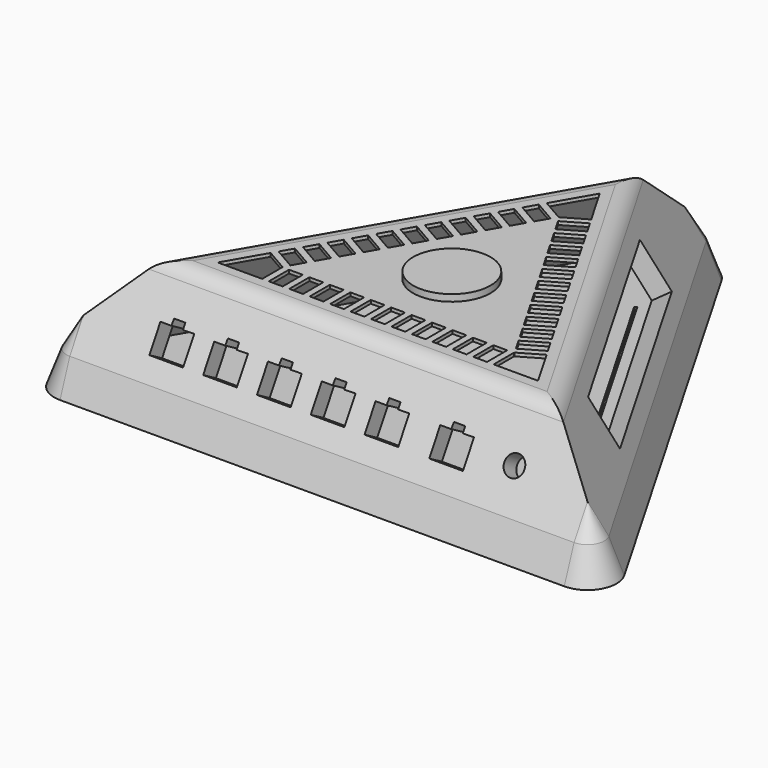
from build123d import *

# Parameters (mm, degrees)
F1_DEPTH      = 25
F1_TAPER      = 30
F1_DEPTH_BACK = 10
F1_TAPER_BACK = -20
F2_R          = 6
F3_R          = 11.5
F4_DEPTH      = 2
F6_R          = 7.5
F7_DEPTH      = 3
F8_R          = 32.5
F9_DEPTH      = 5
F10_R         = 3
F11_DEPTH     = 2
F13_DEPTH     = 5
F15_W         = 1.9796080887
F15_H         = 8.6034480482
F16_DEPTH     = 1
F17_DEPTH     = 10
F19_DEPTH     = 10
F21_DEPTH     = 24
F21_TAPER     = 30


with BuildPart() as f1:
    # F0 (on Top) → F1 (new body, two sides)
    with BuildSketch(Plane.XY) as f1_sk:
        with BuildLine():
            Line((-75, -48.3012701892), (75, -48.3012701892))
            ThreePointArc((75, -48.3012701892), (79.3301270189, -45.8012701892), (79.3301270189, -40.8012701892))
            Line((79.3301270189, -40.8012701892), (4.3301270189, 89.1025403784))
            ThreePointArc((4.3301270189, 89.1025403784), (0, 91.6025403784), (-4.3301270189, 89.1025403784))
            Line((-4.3301270189, 89.1025403784), (-79.3301270189, -40.8012701892))
            ThreePointArc((-79.3301270189, -40.8012701892), (-79.3301270189, -45.8012701892), (-75, -48.3012701892))
        make_face()
    extrude(amount=F1_DEPTH, taper=F1_TAPER)
    extrude(f1_sk.sketch, amount=-F1_DEPTH_BACK, taper=F1_TAPER_BACK)

    # F2
    f2_edges = [f1.edges().sort_by_distance(p)[0] for p in [
        (-29.330127, 16.933757, 25),
        (0, -33.867513, 25),
        (29.330127, 16.933757, 25),
    ]]
    fillet(f2_edges, radius=F2_R)

    # F3 (on face) → F4 (join)
    with BuildSketch(Plane.XY.offset(25)):
        Circle(F3_R)
    extrude(amount=F4_DEPTH)

    # F6 (on face) → F7 (join)
    with BuildSketch(Plane(origin=(0, 0, -10), x_dir=(1, 0, 0), z_dir=(0, 0, -1))):
        with BuildLine():
            ThreePointArc((-57.6663998078, 35.0832771161), (-56.8520972482, 36.9572319185), (-56.5737775642, 38.9814190179))
            ThreePointArc((-56.5737775642, 38.9814190179), (-71.2954578802, 41.0056061173), (-57.6663998078, 35.0832771161))
        make_face()
        with Locations((64.0737775642, 38.9814190179)):
            Circle(F6_R)
        with Locations((0, -75)):
            Circle(F6_R)
    extrude(amount=F7_DEPTH)

    # F8 (on face) → F9 (cut)
    with BuildSketch(Plane(origin=(0, 0, -10), x_dir=(1, 0, 0), z_dir=(0, 0, -1))):
        Circle(F8_R)
    extrude(amount=-F9_DEPTH, mode=Mode.SUBTRACT)

    # F10 (on face) → F11 (cut)
    with BuildSketch(Plane(origin=(0, -36.2259526419, 20.9150635095), x_dir=(1, 0, 0), z_dir=(0, -0.8660254038, 0.5))):
        Polygon((-53.9876961336, -9.3026818497), (-53.9876961336, -17.5021458417), (-43.9876961336, -17.5021458417), (-43.9579116181, -9.2383237345), (-47.2984413058, -9.3026818497), (-47.2984413058, -7.5021458417), (-50.609186478, -7.5021458417), (-50.7396796718, -9.3026818497), align=None)
        Polygon((-34.7396796718, -9.3026818497), (-37.9876961336, -9.3026818497), (-37.9876961336, -17.5021458417), (-27.9876961336, -17.5021458417), (-27.9579116181, -9.2383237345), (-31.2984413058, -9.3026818497), (-31.2984413058, -7.5021458417), (-34.609186478, -7.5021458417), align=None)
        Polygon((-18.7396796718, -9.3026818497), (-21.9876961336, -9.3026818497), (-21.9876961336, -17.5021458417), (-11.9876961336, -17.5021458417), (-11.9579116181, -9.2383237345), (-15.2984413058, -9.3026818497), (-15.2984413058, -7.5021458417), (-18.609186478, -7.5021458417), align=None)
        Polygon((-2.7396796718, -9.3026818497), (-5.9876961336, -9.3026818497), (-5.9876961336, -17.5021458417), (4.0123038664, -17.5021458417), (4.0420883819, -9.2383237345), (0.7015586942, -9.3026818497), (0.7015586942, -7.5021458417), (-2.609186478, -7.5021458417), align=None)
        Polygon((13.2603203282, -9.3026818497), (10.0123038664, -9.3026818497), (10.0123038664, -17.5021458417), (20.0123038664, -17.5021458417), (20.0420883819, -9.2383237345), (16.7015586942, -9.3026818497), (16.7015586942, -7.5021458417), (13.390813522, -7.5021458417), align=None)
        Polygon((32.5083367899, -9.3026819218), (29.2603203282, -9.3026819218), (29.2603203282, -17.5021459138), (39.2603203282, -17.5021459138), (39.2901048437, -9.2383238067), (35.949575156, -9.3026819218), (35.949575156, -7.5021459138), (32.6388299838, -7.5021459138), align=None)
        with Locations((52.4860955775, -12.1968975291)):
            Circle(F10_R)
    extrude(amount=-F11_DEPTH, mode=Mode.SUBTRACT)

    # F3 (on face) → F13 (cut)
    with BuildSketch(Plane.XY.offset(25)):
        Polygon((-47.6313972081, -27.5), (47.6313972081, -27.5), (0, 55), align=None)
        Polygon((0, 40), (34.6410161514, -20), (-34.6410161514, -20), align=None, mode=Mode.SUBTRACT)
    extrude(amount=-F13_DEPTH, mode=Mode.SUBTRACT)

    # F15 (on offset) → F16 (join)
    with BuildSketch(Plane.XY.offset(25)):
        Polygon((-34.415666014, -19.9025444201), (-34.415666014, -19.79204081), (-34.2808202684, -19.79204081), (-33.3725771272, -18.2189175439), (-40.8233816971, -13.9171935197), (-41.8131857415, -15.6315844141), align=None)
        Polygon((-34.2808202684, -19.79204081), (-34.415666014, -19.79204081), (-34.415666014, -19.9025444201), (-34.3623811716, -19.9333084382), align=None)
        Polygon((-32.4360579252, -19.79204081), (-34.2808202684, -19.79204081), (-34.3623811716, -19.9333084382), (-34.415666014, -19.9025444201), (-34.415666014, -28.3954888582), (-32.4360579252, -28.3954888582), align=None)
        with Locations((-27.3458619696, -24.0937648341)):
            Rectangle(F15_W, F15_H)
        with Locations((-21.2658619696, -24.0937648341)):
            Rectangle(F15_W, F15_H)
        with Locations((-15.1858619696, -24.0937648341)):
            Rectangle(F15_W, F15_H)
        with Locations((-9.1058619696, -24.0937648341)):
            Rectangle(F15_W, F15_H)
        with Locations((-3.0258619696, -24.0937648341)):
            Rectangle(F15_W, F15_H)
        with Locations((3.0541380304, -24.0937648341)):
            Rectangle(F15_W, F15_H)
        with Locations((9.1341380304, -24.0937648341)):
            Rectangle(F15_W, F15_H)
        with Locations((15.2141380304, -24.0937648341)):
            Rectangle(F15_W, F15_H)
        with Locations((21.2941380304, -24.0937648341)):
            Rectangle(F15_W, F15_H)
        with Locations((27.3741380304, -24.0937648341)):
            Rectangle(F15_W, F15_H)
        Polygon((34.2808202684, -19.79204081), (34.4439420748, -19.79204081), (34.4439420748, -19.8535688462), (41.7990477111, -15.6070966271), (40.8092436667, -13.8927057328), (33.3584390968, -18.1944297569), align=None)
        Polygon((34.4439420748, -19.8535688462), (34.4439420748, -19.79204081), (34.2808202684, -19.79204081), (34.3482431412, -19.9088206513), align=None)
        Polygon((34.4439420748, -28.3954888582), (34.4439420748, -19.8535688462), (34.3482431412, -19.9088206513), (34.2808202684, -19.79204081), (32.464333986, -19.79204081), (32.464333986, -28.3954888582), align=None)
        Polygon((25.6092436667, 12.4344665423), (18.1584390968, 8.1327425182), (19.1482431412, 6.4183516238), (26.5990477111, 10.7200756479), align=None)
        Polygon((22.5692436667, 17.6999009973), (15.1184390968, 13.3981769732), (16.1082431412, 11.6837860788), (23.5590477111, 15.9855101029), align=None)
        Polygon((10.4092436667, 38.7616388173), (2.9584390968, 34.4599147932), (3.9482431412, 32.7455238988), (11.3990477111, 37.047247923), align=None)
        Polygon((19.5292436667, 22.9653354523), (12.0784390968, 18.6636114282), (13.0682431412, 16.9492205338), (20.5190477111, 21.2509445579), align=None)
        Polygon((0, 39.58408162), (-0.0815609032, 39.7253492482), (-0.0282760608, 39.7561132663), (-7.3833816971, 44.0025854854), (-8.3731857415, 42.288194591), (-0.9223811716, 37.9864705669), align=None)
        Polygon((-0.0282760608, 39.7561132663), (-0.0815609032, 39.7253492482), (0, 39.58408162), (0.0674228728, 39.7008614612), align=None)
        Polygon((7.3692436667, 44.0270732723), (-0.0282760608, 39.7561132663), (0.0674228728, 39.7008614612), (0, 39.58408162), (0.9082431412, 38.0109583539), (8.3590477111, 42.312682378), align=None)
        Polygon((9.0384390968, 23.9290458832), (10.0282431412, 22.2146549888), (17.4790477111, 26.5163790129), (16.4892436667, 28.2307699073), align=None)
        Polygon((31.6892436667, 1.9035976323), (24.2384390968, -2.3981263918), (25.2282431412, -4.1125172862), (32.6790477111, 0.1892067379), align=None)
        Polygon((27.2784390968, -7.6635608469), (28.2682431412, -9.3779517412), (35.7190477111, -5.0762277171), (34.7292436667, -3.3618368227), align=None)
        Polygon((30.3184390968, -12.9289953019), (31.3082431412, -14.6433861962), (38.7590477111, -10.3416621721), (37.7692436667, -8.6272712777), align=None)
        Polygon((21.1984390968, 2.8673080632), (22.1882431412, 1.1529171688), (29.6390477111, 5.4546411929), (28.6492436667, 7.1690320873), align=None)
        Polygon((5.9984390968, 29.1944803382), (6.9882431412, 27.4800894438), (14.4390477111, 31.7818134679), (13.4492436667, 33.4962043623), align=None)
        Polygon((-23.5731857415, 15.9610223159), (-16.1223811716, 11.6592982918), (-15.1325771272, 13.3736891862), (-22.5833816971, 17.6754132103), align=None)
        Polygon((-26.6131857415, 10.6955878609), (-19.1623811716, 6.3938638368), (-18.1725771272, 8.1082547312), (-25.6233816971, 12.4099787553), align=None)
        Polygon((-38.7731857415, -10.3661499591), (-31.3223811716, -14.6678739832), (-30.3325771272, -12.9534830889), (-37.7833816971, -8.6517590647), align=None)
        Polygon((-29.6531857415, 5.4301534059), (-22.2023811716, 1.1284293818), (-21.2125771272, 2.8428202762), (-28.6633816971, 7.1445443003), align=None)
        Polygon((-25.2423811716, -4.1370050732), (-24.2525771272, -2.4226141788), (-31.7033816971, 1.8791098453), (-32.6931857415, 0.1647189509), align=None)
        Polygon((-17.4931857415, 26.491891226), (-10.0423811716, 22.1901672018), (-9.0525771272, 23.9045580962), (-16.5033816971, 28.2062821203), align=None)
        Polygon((-7.0023811716, 27.4556016568), (-6.0125771272, 29.1699925512), (-13.4633816971, 33.4717165753), (-14.4531857415, 31.757325681), align=None)
        Polygon((-3.9623811716, 32.7210361119), (-2.9725771272, 34.4354270062), (-10.4233816971, 38.7371510303), (-11.4131857415, 37.022760136), align=None)
        Polygon((-13.0823811716, 16.9247327468), (-12.0925771272, 18.6391236412), (-19.5433816971, 22.9408476653), (-20.5331857415, 21.2264567709), align=None)
        Polygon((-28.2823811716, -9.4024395282), (-27.2925771272, -7.6880486338), (-34.7433816971, -3.3863246097), (-35.7331857415, -5.1007155041), align=None)
    extrude(amount=-F16_DEPTH)

    # F10 (on face) → F17 (cut)
    with BuildSketch(Plane(origin=(0, -36.2259526419, 20.9150635095), x_dir=(1, 0, 0), z_dir=(0, -0.8660254038, 0.5))):
        Polygon((-53.9876961336, -9.3026818497), (-53.9876961336, -17.5021458417), (-43.9876961336, -17.5021458417), (-43.9579116181, -9.2383237345), (-47.2984413058, -9.3026818497), (-47.2984413058, -7.5021458417), (-50.609186478, -7.5021458417), (-50.7396796718, -9.3026818497), align=None)
        Polygon((-34.7396796718, -9.3026818497), (-37.9876961336, -9.3026818497), (-37.9876961336, -17.5021458417), (-27.9876961336, -17.5021458417), (-27.9579116181, -9.2383237345), (-31.2984413058, -9.3026818497), (-31.2984413058, -7.5021458417), (-34.609186478, -7.5021458417), align=None)
        Polygon((-18.7396796718, -9.3026818497), (-21.9876961336, -9.3026818497), (-21.9876961336, -17.5021458417), (-11.9876961336, -17.5021458417), (-11.9579116181, -9.2383237345), (-15.2984413058, -9.3026818497), (-15.2984413058, -7.5021458417), (-18.609186478, -7.5021458417), align=None)
        Polygon((-2.7396796718, -9.3026818497), (-5.9876961336, -9.3026818497), (-5.9876961336, -17.5021458417), (4.0123038664, -17.5021458417), (4.0420883819, -9.2383237345), (0.7015586942, -9.3026818497), (0.7015586942, -7.5021458417), (-2.609186478, -7.5021458417), align=None)
        Polygon((13.2603203282, -9.3026818497), (10.0123038664, -9.3026818497), (10.0123038664, -17.5021458417), (20.0123038664, -17.5021458417), (20.0420883819, -9.2383237345), (16.7015586942, -9.3026818497), (16.7015586942, -7.5021458417), (13.390813522, -7.5021458417), align=None)
        Polygon((32.5083367899, -9.3026819218), (29.2603203282, -9.3026819218), (29.2603203282, -17.5021459138), (39.2603203282, -17.5021459138), (39.2901048437, -9.2383238067), (35.949575156, -9.3026819218), (35.949575156, -7.5021459138), (32.6388299838, -7.5021459138), align=None)
        with Locations((52.4860955775, -12.1968975291)):
            Circle(F10_R)
    extrude(amount=-F17_DEPTH, mode=Mode.SUBTRACT)

    # F18 (on face) → F19 (cut)
    with BuildSketch(Plane(origin=(31.3725952642, 18.112976321, 20.9150635095), x_dir=(-0.3602883461, 0.9013878189, -0.2401922307), z_dir=(0.75, 0.4330127019, 0.5))):
        Polygon((39.4700496493, 7.4937882787), (-37.3914641771, -14.6942195703), (-33.2312127054, -29.1057534127), (43.630301121, -6.9177455637), align=None)
    extrude(amount=-F19_DEPTH, mode=Mode.SUBTRACT)

    # F20 (on Top) → F21 (cut)
    with BuildSketch(Plane.XY):
        Polygon((-72.7461339179, -42), (72.7461339179, -42), (0, 84), align=None)
    extrude(amount=F21_DEPTH, taper=F21_TAPER, mode=Mode.SUBTRACT)


solid = f1.part
